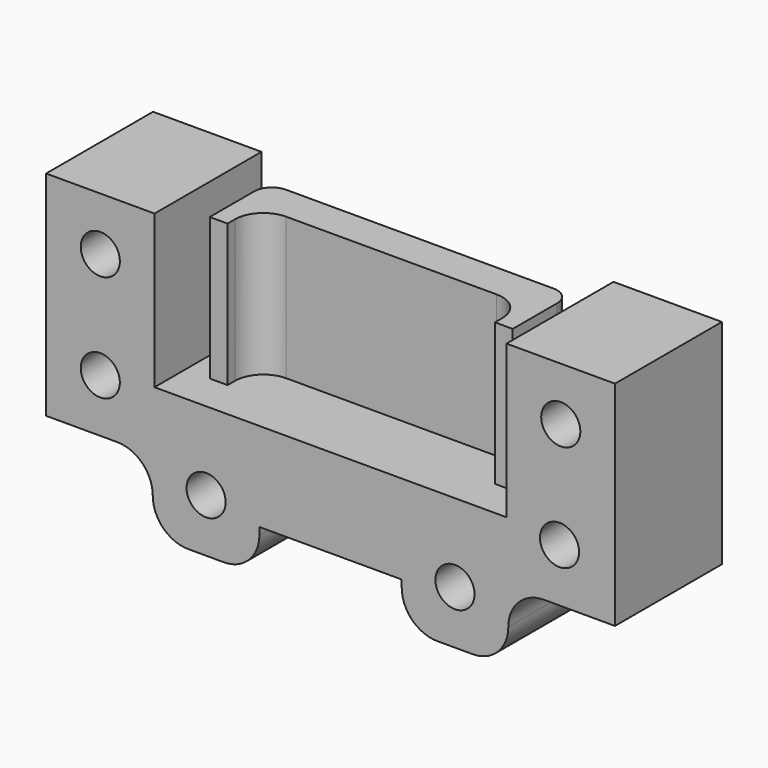
from build123d import *

# Parameters (mm, degrees)
F1_DEPTH = 18.8
F3_DEPTH = 20
F4_R     = 4
F5_R     = 2.5
F6_R     = 2.5
F8_R     = 4.99999
F12_D    = 5.5


# Not quite as in the source:
# - two fillets or chamfers of one size are made in one step
# - a fillet or chamfer is up to 0.001 mm smaller than in the source, because OpenCascade refuses the exact size


with BuildPart() as f1:
    # F0 (on Front) → F1 (new body)
    with BuildSketch(Plane.XZ):
        Polygon((-24.75, 21.5), (-40, 21.5), (-40, -8.5), (-25, -8.5), (-25, -18.5), (-10, -18.5), (-10, -12.5), (10.0144529715, -12.5), (10.0144529715, -18.5), (25, -18.5), (25, -8.5), (40, -8.5), (40, 21.5), (24.75, 21.5), (24.75, 0), (-24.75, 0), align=None)
    extrude(amount=F1_DEPTH)

    # F8 (radius 5 in the source; OpenCascade refuses exactly that, so slightly less here)
    f8_edges = [f1.edges().sort_by_distance(p)[0] for p in [
        (-25, -9.4, -18.5),
        (25, -9.4, -18.5),
        (-25, -9.4, -8.5),
        (-10, -9.4, -18.5),
        (10.014453, -9.4, -18.5),
        (25, -9.4, -8.5),
    ]]
    fillet(f8_edges, radius=F8_R)

    # F12 (through all)
    with Locations(Plane.XZ.offset(18.8)):
        with Locations((-32.375, 14), (-32.375, -1), (-17.5, -11), (17.5, -11), (32.2044789791, -1), (32.375, 14)):
            Hole(F12_D / 2)


with BuildPart() as f3:
    # F2 (on face) → F3 (new body)
    with BuildSketch(Plane.XY):
        Polygon((21.3, -3.1), (-21.3, -3.1), (-21.3, -13.4), (-18.8, -13.4), (-18.8, -8.1), (18.8, -8.1), (18.8, -13.4), (21.3, -13.4), align=None)
    extrude(amount=F3_DEPTH)

    # F4
    f4_edges = [f3.edges().sort_by_distance(p)[0] for p in [
        (-18.8, -8.1, 10),
        (18.8, -8.1, 10),
    ]]
    fillet(f4_edges, radius=F4_R)

    # F5
    f5_edges = [f3.edges().sort_by_distance(p)[0] for p in [
        (21.3, -3.1, 10),
    ]]
    fillet(f5_edges, radius=F5_R)

    # F6
    f6_edges = [f3.edges().sort_by_distance(p)[0] for p in [
        (-21.3, -3.1, 10),
    ]]
    fillet(f6_edges, radius=F6_R)


solid = Compound([f1.part, f3.part])
